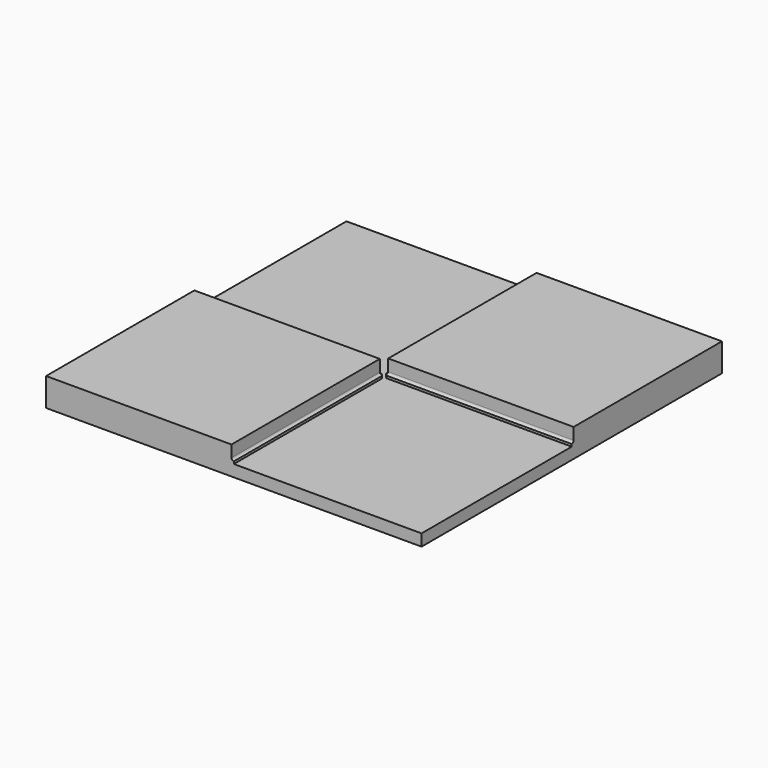
from build123d import *

# Parameters (mm, degrees)
F0_W     = 508
F0_H     = 508
F1_DEPTH = 38.1
F2_W     = 250.825
F2_H     = 250.825
F2_H_2   = 6.35
F2_W_2   = 6.35
F3_DEPTH = 19.05
F4_R     = 3.17499
F6_DEPTH = 22.225


# Not quite as in the source:
# - a fillet or chamfer is up to 0.001 mm smaller than in the source, because OpenCascade refuses the exact size
# - a pattern or mirror of a feature is missing from the dataset's text; its kind, count and spacing are read off the source's solid


with BuildPart() as f1:
    # F0 (on Top) → F1 (new body)
    with BuildSketch(Plane.XY):
        Rectangle(F0_W, F0_H)
    extrude(amount=F1_DEPTH)

    # F2 (on face) → F3 (cut)
    with BuildSketch(Plane.XY.offset(38.1)):
        with Locations((128.5875, -128.5875)):
            Rectangle(F2_W, F2_H)
        with Locations((128.5875, 0)):
            Rectangle(F2_W, F2_H_2)
        with Locations((0, -128.5875)):
            Rectangle(F2_W_2, F2_H)
        Rectangle(F2_W_2, F2_H_2)
        with Locations((-128.5875, 0)):
            Rectangle(F2_W, F2_H_2)
        with Locations((0, 128.5875)):
            Rectangle(F2_W_2, F2_H)
    extrude(amount=-F3_DEPTH, mode=Mode.SUBTRACT)

    # F4 (radius 3.175 in the source; OpenCascade refuses exactly that, so slightly less here)
    f4_edges = [f1.edges().sort_by_distance(p)[0] for p in [
        (-128.5875, -3.175, 19.05),
        (-3.175, -128.5875, 19.05),
        (3.175, 128.5875, 19.05),
        (128.5875, 3.175, 19.05),
        (-3.175, 128.5875, 19.05),
        (-128.5875, 3.175, 19.05),
    ]]
    fillet(f4_edges, radius=F4_R)

    # F5 (on face) → F6 (cut)
    with BuildSketch(Plane.XY.offset(38.1)):
        Polygon((0, 254), (-254, 254), (-254, 0), (-3.3675960454, 0), (-1.6837980227, -1.6837980227), (1.6837980227, 1.6837980227), (0, 3.3675960454), align=None)
    f6 = extrude(amount=-F6_DEPTH, mode=Mode.SUBTRACT)

    # F6_copies: F6 across plane
    add(f6.mirror(Plane(origin=(0, 0, 0), x_dir=(-0.7071067812, -0.7071067812, 0), z_dir=(0.7071067812, -0.7071067812, 0))), mode=Mode.SUBTRACT)


solid = f1.part
